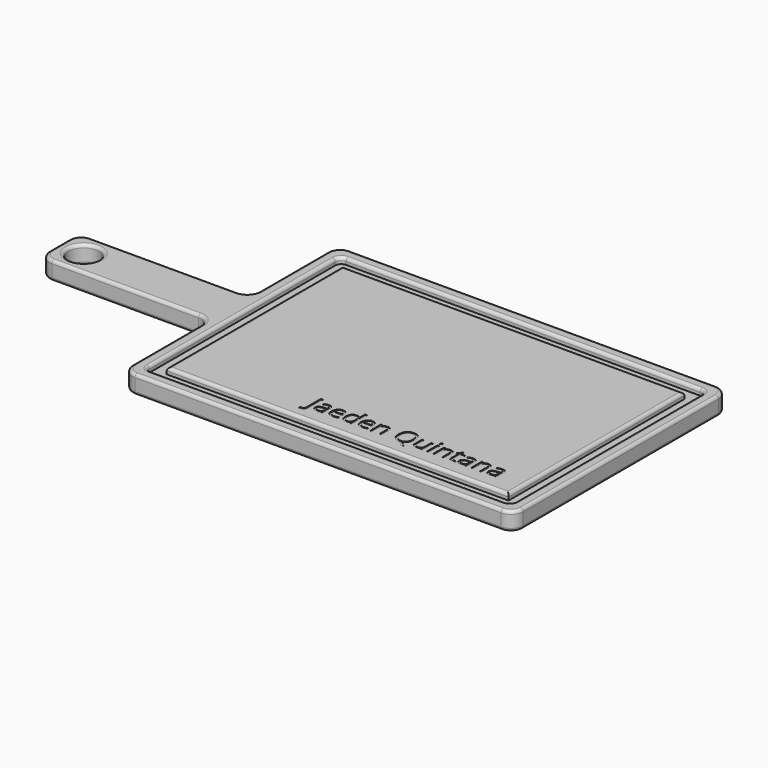
from build123d import *

# Parameters (mm, degrees)
F0_W          = 177.8
F0_H          = 50.8
F1_DEPTH      = 19.05
F2_R          = 15.875
F3_DEPTH      = 25.4
F5_DEPTH      = 6.35
F6_R          = 6.35
F7_R          = 12.7
F8_R          = 12.7
F9_R          = 3.175
F10_TEXT_SIZE = 25.9452557657
F11_DEPTH     = 0.508


# Not quite as in the source:
# - Text() gives the source's letters only with a copy of the font that has no kerning and outlines rounded to 1/6400 em; it was checked with that copy


with BuildPart() as f1:
    # F0 (on Top) → F1 (new body)
    with BuildSketch(Plane.XY):
        Polygon((0, 114.3), (0, 0), (406.4, 0), (406.4, 279.4), (0, 279.4), (0, 165.1), align=None)
        with Locations((-88.9, 139.7)):
            Rectangle(F0_W, F0_H)
    extrude(amount=F1_DEPTH)

    # F2 (on face) → F3 (cut)
    with BuildSketch(Plane.XY.offset(19.05)):
        with Locations((-152.4, 139.7)):
            Circle(F2_R)
    extrude(amount=-F3_DEPTH, mode=Mode.SUBTRACT)

    # F4 (on face) → F5 (cut)
    with BuildSketch(Plane.XY.offset(19.05)):
        Polygon((12.7000004292, 114.3), (12.7000004292, 12.7000004292), (393.6999995708, 12.7000004292), (393.6999995708, 266.6999995708), (12.7000004292, 266.6999995708), (12.7000004292, 165.1), align=None)
        Polygon((25.3999918938, 114.3), (25.3999918938, 165.1), (25.3999918938, 254.0000081062), (381.0000081062, 254.0000081062), (381.0000081062, 25.3999918938), (25.3999918938, 25.3999918938), align=None, mode=Mode.SUBTRACT)
    extrude(amount=-F5_DEPTH, mode=Mode.SUBTRACT)

    # F6
    f6_edges = [f1.edges().sort_by_distance(p)[0] for p in [
        (12.7, 266.7, 15.875),
        (393.7, 266.7, 15.875),
        (393.7, 12.7, 15.875),
        (12.7, 12.7, 15.875),
    ]]
    fillet(f6_edges, radius=F6_R)

    # F7
    f7_edges = [f1.edges().sort_by_distance(p)[0] for p in [
        (-177.8, 114.3, 9.525),
        (-177.8, 165.1, 9.525),
    ]]
    fillet(f7_edges, radius=F7_R)

    # F8
    f8_edges = [f1.edges().sort_by_distance(p)[0] for p in [
        (0, 279.4, 9.525),
        (0, 165.1, 9.525),
        (406.4, 279.4, 9.525),
        (406.4, 0, 9.525),
        (0, 0, 9.525),
        (0, 114.3, 9.525),
    ]]
    fillet(f8_edges, radius=F8_R)

    # F9
    f9_edges = [f1.edges().sort_by_distance(p)[0] for p in [
        (203.2, 254.000008, 19.05),
        (381.000008, 139.7, 19.05),
        (203.2, 25.399992, 19.05),
        (25.399992, 139.7, 19.05),
        (-88.9, 114.3, 19.05),
        (-3.719744, 110.580256, 19.05),
        (-174.080256, 118.019744, 19.05),
        (0, 57.15, 19.05),
        (-177.8, 139.7, 19.05),
        (3.719744, 3.719744, 19.05),
        (-174.080256, 161.380256, 19.05),
        (203.2, 0, 19.05),
        (-88.9, 165.1, 19.05),
        (402.680256, 3.719744, 19.05),
        (-3.719744, 168.819744, 19.05),
        (406.4, 139.7, 19.05),
        (0, 222.25, 19.05),
        (402.680256, 275.680256, 19.05),
        (3.719744, 275.680256, 19.05),
        (203.2, 279.4, 19.05),
        (203.2, 12.7, 19.05),
        (14.559872, 14.559872, 19.05),
        (391.840128, 14.559872, 19.05),
        (12.7, 139.7, 19.05),
        (393.7, 139.7, 19.05),
        (14.559872, 264.840128, 19.05),
        (391.840128, 264.840128, 19.05),
        (203.2, 266.7, 19.05),
        (-168.275, 139.7, 19.05),
        (203.2, 0, 0),
        (12.7, 0, 9.525),
        (393.7, 0, 9.525),
        (-88.9, 114.3, 0),
        (-3.719744, 110.580256, 0),
        (-174.080256, 118.019744, 0),
        (0, 57.15, 0),
        (-177.8, 139.7, 0),
        (3.719744, 3.719744, 0),
        (-174.080256, 161.380256, 0),
        (-88.9, 165.1, 0),
        (402.680256, 3.719744, 0),
        (-3.719744, 168.819744, 0),
        (406.4, 139.7, 0),
        (0, 222.25, 0),
        (402.680256, 275.680256, 0),
        (3.719744, 275.680256, 0),
        (203.2, 279.4, 0),
        (-168.275, 139.7, 0),
    ]]
    fillet(f9_edges, radius=F9_R)

    # F10 (on face) → F11 (cut)
    with BuildSketch(Plane.XY.offset(19.05)):
        with Locations((155.426451306, 41.8522218053)):
            Text('Jaeden Quintana', F10_TEXT_SIZE, font='Open Sans', text_align=(TextAlign.LEFT, TextAlign.BOTTOM))
    extrude(amount=-F11_DEPTH, mode=Mode.SUBTRACT)


solid = f1.part
